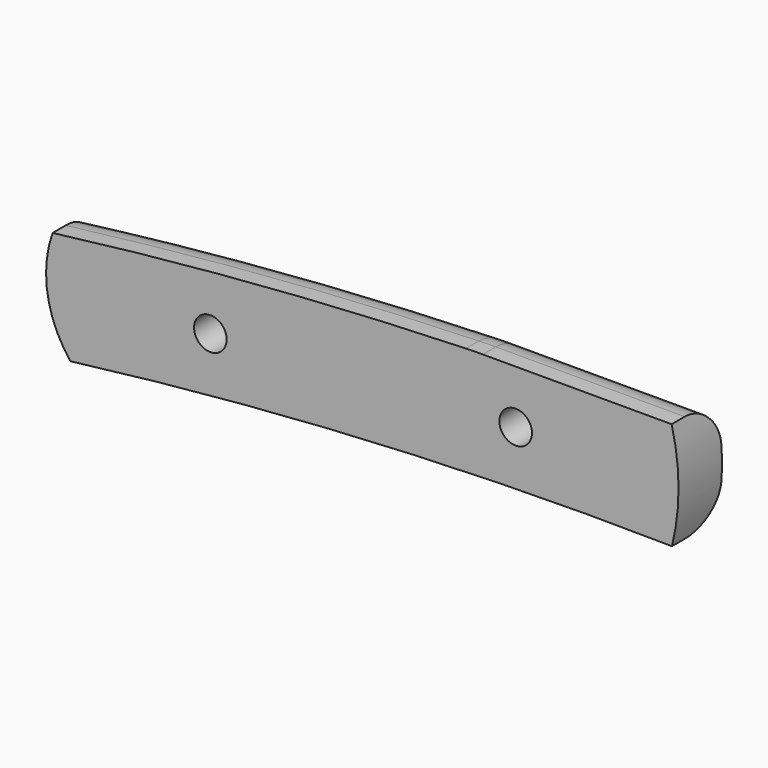
from build123d import *

# Parameters (mm, degrees)
F0_R         = 3
F1_DEPTH     = 10
F2_T3_ANGLE  = 6.7239804363
F2_T6_ANGLE  = 10.729424982
F2_T9_DEPTH  = 52.3011751173
F2_T12_ANGLE = 1.7828949869


# Not quite as in the source:
# - a fillet or chamfer that OpenCascade refuses, or shapes differently, is made with other operations: its cross-section is extruded or revolved along the edge and cut away or added


with BuildPart() as f1:
    # F0 (on Front) → F1 (new body)
    with BuildSketch(Plane.XZ):
        with BuildLine():
            ThreePointArc((16.7161625637, 9.1005522793), (15.1603559483, 9.0884488757), (13.604925944, 9.0521415948))
            ThreePointArc((13.604925944, 9.0521415948), (-24.5259537531, 6.9533029462), (-62.5132279063, 3.0371680453))
            ThreePointArc((-62.5132279063, 3.0371680453), (-63.4446975244, -7.2627028514), (-59.2295458713, -16.7066147888))
            ThreePointArc((-59.2295458713, -16.7066147888), (-3.9332598443, -11.7153648591), (51.5779973344, -10.6703047235))
            ThreePointArc((51.5779973344, -10.6703047235), (52.7884384629, -0.7810693697), (51.517337681, 9.1005522793))
            Line((51.517337681, 9.1005522793), (16.7161625637, 9.1005522793))
        make_face()
        with Locations((-33.4603461426, -3.8443253384)):
            Circle(F0_R, mode=Mode.SUBTRACT)
        with Locations((22.7880547631, -0.7167291473)):
            Circle(F0_R, mode=Mode.SUBTRACT)
    extrude(amount=F1_DEPTH)

    # F2: fillet of radius 7 on 4 edges, made by hand


with BuildPart() as f2_tool1:
    # F2_s2 → F2_t3 (revolve)
    with BuildSketch(Plane(origin=(13.8732538603, 0, 0.4318388106), x_dir=(0, 1, 0), z_dir=(0.9995158932, 0, 0.0311123662))):
        with BuildLine():
            ThreePointArc((-7, 8.624477953), (-2.0502525317, 6.5742254213), (0, 1.624477953))
            Line((0, 1.624477953), (0, 8.624477953))
            Line((0, 8.624477953), (-7, 8.624477953))
        make_face()
    revolve(axis=Axis((38.4948189015, 0, -790.5605729296), (0, -1, 0)), revolution_arc=F2_T3_ANGLE)


with BuildPart() as f2_tool4:
    # F2_s5 → F2_t6 (revolve)
    with BuildSketch(Plane(origin=(-77.6853434409, 0, -11.5863862591), x_dir=(0, 1, 0), z_dir=(-0.9890600521, 0, -0.1475134342))):
        with BuildLine():
            ThreePointArc((-7, 7.5903844134), (-2.0502525317, 5.5401318817), (0, 0.5903844134))
            Line((0, 0.5903844134), (0, 7.5903844134))
            Line((0, 7.5903844134), (-7, 7.5903844134))
        make_face()
    revolve(axis=Axis((38.4948189015, 0, -790.5605729293), (0, 1, 0)), revolution_arc=F2_T6_ANGLE)


with BuildPart() as f2_tool7:
    # F2_s8 → F2_t9 (new body)
    with BuildSketch(Plane.YZ.offset(69.017337681)):
        with BuildLine():
            ThreePointArc((-7, 9.1005522793), (-2.0502525317, 7.0502997476), (0, 2.1005522793))
            Line((0, 2.1005522793), (0, 9.1005522793))
            Line((0, 9.1005522793), (-7, 9.1005522793))
        make_face()
    extrude(amount=-F2_T9_DEPTH)


with BuildPart() as f2_tool10:
    # F2_s11 → F2_t12 (revolve)
    with BuildSketch(Plane.YZ.offset(16.7161625637)):
        with BuildLine():
            ThreePointArc((-7, 9.1005522793), (-2.0502525317, 7.0502997476), (0, 2.1005522793))
            Line((0, 2.1005522793), (0, 9.1005522793))
            Line((0, 9.1005522793), (-7, 9.1005522793))
        make_face()
    revolve(axis=Axis((16.7161625637, 0, -90.8994477206), (0, -1, 0)), revolution_arc=F2_T12_ANGLE)


with BuildPart() as f1_1:
    add(f1.part)

    # F2_t13: cut F2_tool1, F2_tool4, F2_tool7, F2_tool10
    add([f2_tool1.part, f2_tool4.part, f2_tool7.part, f2_tool10.part], mode=Mode.SUBTRACT)


solid = f1_1.part
